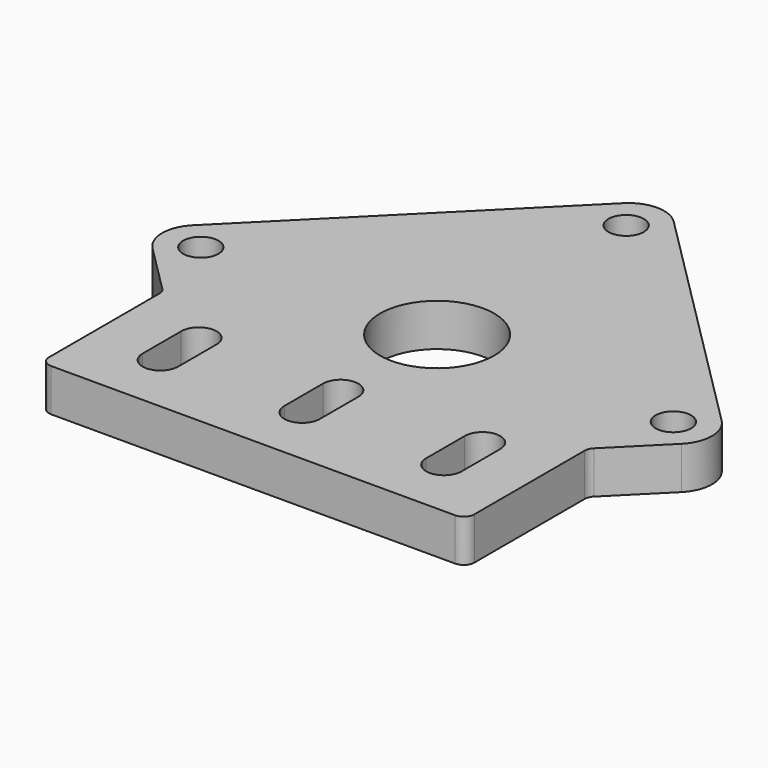
from build123d import *

# Parameters (mm, degrees)
F0_R     = 4.6
F0_R_2   = 8.05
F0_R_3   = 2.5
F1_DEPTH = 6


# Not quite as in the source:
# - ends of sketch curves that miss each other by under 0.0002 mm in the source are joined


with BuildPart() as f1:
    # F0 (on Top) → F1 (new body)
    with BuildSketch(Plane.XY):
        with BuildLine():
            ThreePointArc((-30, -34.104246), (-29.5606601718, -35.1649061718), (-28.5, -35.604246))
            Line((-28.5, -35.604246), (28.5, -35.604246))
            ThreePointArc((28.5, -35.604246), (29.5606601718, -35.1649061718), (30, -34.104246))
            Line((30, -34.104246), (30, -14.645125))
            ThreePointArc((30, -14.645125), (30.1141807012, -14.0710998515), (30.4393398282, -13.5844648282))
            Line((30.4393398282, -13.5844648282), (37.314025, -6.70978))
            ThreePointArc((37.314025, -6.70978), (38.778491, -3.174246), (37.3140249059, 0.3612879059))
            Line((37.3140249059, 0.3612879059), (3.535534, 34.139779))
            ThreePointArc((3.535534, 34.139779), (0, 35.604245), (-3.5355339059, 34.1397789059))
            Line((-3.5355339059, 34.1397789059), (-37.314025, 0.361288))
            ThreePointArc((-37.314025, 0.361288), (-38.778491, -3.174246), (-37.3140249059, -6.7097799059))
            Line((-37.3140249059, -6.7097799059), (-30.43934, -13.584465))
            ThreePointArc((-30.43934, -13.584465), (-30.1141807012, -14.0710998515), (-30, -14.645125))
            Line((-30, -14.645125), (-30, -34.104246))
        make_face()
        with BuildLine():
            ThreePointArc((-24.6, -20.174246), (-20, -15.574246), (-15.4, -20.174246))
            Line((-15.4, -20.174246), (-15.4, -26.974246))
            ThreePointArc((-15.4, -26.974246), (-20, -31.574246), (-24.6, -26.974246))
            Line((-24.6, -26.974246), (-24.6, -20.174246))
        make_face(mode=Mode.SUBTRACT)
        with Locations((-33.333, -3.174246)):
            Circle(F0_R, mode=Mode.SUBTRACT)
        with BuildLine():
            ThreePointArc((4.6, -26.974246), (0, -31.574246), (-4.6, -26.974246))
            Line((-4.6, -26.974246), (-4.6, -20.174246))
            ThreePointArc((-4.6, -20.174246), (0, -15.574246), (4.6, -20.174246))
            Line((4.6, -20.174246), (4.6, -26.974246))
        make_face(mode=Mode.SUBTRACT)
        with BuildLine():
            ThreePointArc((24.6, -26.974246), (20, -31.574246), (15.4, -26.974246))
            Line((15.4, -26.974246), (15.4, -20.174246))
            ThreePointArc((15.4, -20.174246), (20, -15.574246), (24.6, -20.174246))
            Line((24.6, -20.174246), (24.6, -26.974246))
        make_face(mode=Mode.SUBTRACT)
        with Locations((0, -3.174246)):
            Circle(F0_R_2, mode=Mode.SUBTRACT)
        with Locations((33.333, -3.174246)):
            Circle(F0_R, mode=Mode.SUBTRACT)
        with Locations((0, 30.158782)):
            Circle(F0_R, mode=Mode.SUBTRACT)
        with Locations((-33.333, -3.174246)):
            Circle(F0_R)
        with Locations((-33.333, -3.174246)):
            Circle(F0_R_3, mode=Mode.SUBTRACT)
        with Locations((0, 30.158782)):
            Circle(F0_R)
        with Locations((0, 30.158782)):
            Circle(F0_R_3, mode=Mode.SUBTRACT)
        with Locations((33.333, -3.174246)):
            Circle(F0_R)
        with Locations((33.333, -3.174246)):
            Circle(F0_R_3, mode=Mode.SUBTRACT)
        with BuildLine():
            Line((15.4, -20.174246), (15.4, -26.974246))
            ThreePointArc((15.4, -26.974246), (20, -31.574246), (24.6, -26.974246))
            Line((24.6, -26.974246), (24.6, -20.174246))
            ThreePointArc((24.6, -20.174246), (20, -15.574246), (15.4, -20.174246))
        make_face()
        with BuildLine():
            ThreePointArc((22.5, -26.974246), (20, -29.474246), (17.5, -26.974246))
            Line((17.5, -26.974246), (17.5, -20.174246))
            ThreePointArc((17.5, -20.174246), (20, -17.674246), (22.5, -20.174246))
            Line((22.5, -20.174246), (22.5, -26.974246))
        make_face(mode=Mode.SUBTRACT)
        with BuildLine():
            Line((-4.6, -20.174246), (-4.6, -26.974246))
            ThreePointArc((-4.6, -26.974246), (0, -31.574246), (4.6, -26.974246))
            Line((4.6, -26.974246), (4.6, -20.174246))
            ThreePointArc((4.6, -20.174246), (0, -15.574246), (-4.6, -20.174246))
        make_face()
        with BuildLine():
            ThreePointArc((2.5, -26.974246), (0, -29.474246), (-2.5, -26.974246))
            Line((-2.5, -26.974246), (-2.5, -20.174246))
            ThreePointArc((-2.5, -20.174246), (0, -17.674246), (2.5, -20.174246))
            Line((2.5, -20.174246), (2.5, -26.974246))
        make_face(mode=Mode.SUBTRACT)
        with BuildLine():
            Line((-15.4, -26.974246), (-15.4, -20.174246))
            ThreePointArc((-15.4, -20.174246), (-20, -15.574246), (-24.6, -20.174246))
            Line((-24.6, -20.174246), (-24.6, -26.974246))
            ThreePointArc((-24.6, -26.974246), (-20, -31.574246), (-15.4, -26.974246))
        make_face()
        with BuildLine():
            ThreePointArc((-17.5, -26.974246), (-20, -29.474246), (-22.5, -26.974246))
            Line((-22.5, -26.974246), (-22.5, -20.174246))
            ThreePointArc((-22.5, -20.174246), (-20, -17.674246), (-17.5, -20.174246))
            Line((-17.5, -20.174246), (-17.5, -26.974246))
        make_face(mode=Mode.SUBTRACT)
    extrude(amount=F1_DEPTH)


solid = f1.part
